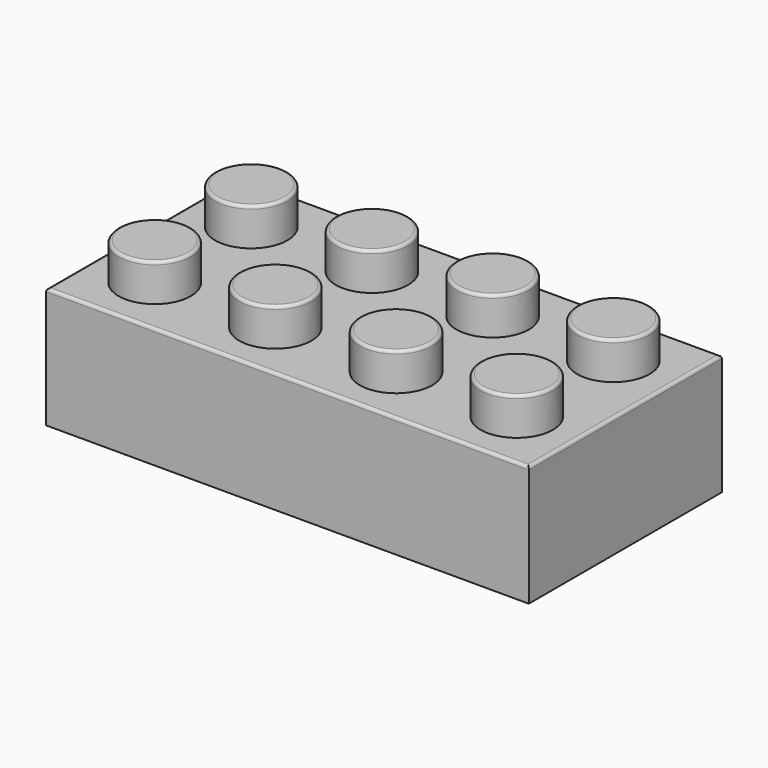
from build123d import *

# Parameters (mm, degrees)
F0_W     = 160
F0_H     = 80
F1_DEPTH = 40
F2_W     = 144.0218614806
F2_H     = 64.0218614806
F3_DEPTH = 30
F5_R     = 1
F4_R     = 12
F6_DEPTH = 12.44405
F7_R     = 1
F8_R     = 1
F9_R     = 1
F10_R    = 1
F11_R    = 1
F12_R    = 1
F13_R    = 1
F14_R    = 1


with BuildPart() as f1:
    # F0 (on Top) → F1 (new body)
    with BuildSketch(Plane.XY):
        with Locations((15.6917236745, 5.7171181207)):
            Rectangle(F0_W, F0_H)
    extrude(amount=F1_DEPTH)

    # F2 (on face) → F3 (cut)
    with BuildSketch(Plane(origin=(0, 0, 0), x_dir=(1, 0, 0), z_dir=(0, 0, -1))):
        with Locations((15.6917236745, -5.7171181207)):
            Rectangle(F2_W, F2_H)
    extrude(amount=-F3_DEPTH, mode=Mode.SUBTRACT)

    # F5
    f5_edges = [f1.edges().sort_by_distance(p)[0] for p in [
        (15.691724, 45.717118, 40),
        (-64.308276, 5.717118, 40),
        (15.691724, -34.282882, 40),
        (95.691724, 5.717118, 40),
    ]]
    fillet(f5_edges, radius=F5_R)

    # F4 (on face) → F6 (join)
    with BuildSketch(Plane.XY.offset(40)):
        with Locations((-44.3082763255, -14.2828818793)):
            Circle(F4_R)
        with Locations((-4.3082763255, -14.2828818793)):
            Circle(F4_R)
        with Locations((35.6917236745, -14.2828818793)):
            Circle(F4_R)
        with Locations((75.6917236745, -14.2828818793)):
            Circle(F4_R)
        with Locations((75.6917236745, 25.7171181207)):
            Circle(F4_R)
        with Locations((35.6917236745, 25.7171181207)):
            Circle(F4_R)
        with Locations((-4.3082763255, 25.7171181207)):
            Circle(F4_R)
        with Locations((-44.3082763255, 25.7171181207)):
            Circle(F4_R)
    extrude(amount=F6_DEPTH)

    # F7
    f7_edges = [f1.edges().sort_by_distance(p)[0] for p in [
        (-56.308276, 25.717118, 52.44405),
    ]]
    fillet(f7_edges, radius=F7_R)

    # F8
    f8_edges = [f1.edges().sort_by_distance(p)[0] for p in [
        (-16.308276, 25.717118, 52.44405),
    ]]
    fillet(f8_edges, radius=F8_R)

    # F9
    f9_edges = [f1.edges().sort_by_distance(p)[0] for p in [
        (23.691724, 25.717118, 52.44405),
    ]]
    fillet(f9_edges, radius=F9_R)

    # F10
    f10_edges = [f1.edges().sort_by_distance(p)[0] for p in [
        (63.691724, 25.717118, 52.44405),
    ]]
    fillet(f10_edges, radius=F10_R)

    # F11
    f11_edges = [f1.edges().sort_by_distance(p)[0] for p in [
        (-56.308276, -14.282882, 52.44405),
    ]]
    fillet(f11_edges, radius=F11_R)

    # F12
    f12_edges = [f1.edges().sort_by_distance(p)[0] for p in [
        (-16.308276, -14.282882, 52.44405),
    ]]
    fillet(f12_edges, radius=F12_R)

    # F13
    f13_edges = [f1.edges().sort_by_distance(p)[0] for p in [
        (23.691724, -14.282882, 52.44405),
    ]]
    fillet(f13_edges, radius=F13_R)

    # F14
    f14_edges = [f1.edges().sort_by_distance(p)[0] for p in [
        (63.691724, -14.282882, 52.44405),
    ]]
    fillet(f14_edges, radius=F14_R)


solid = f1.part
